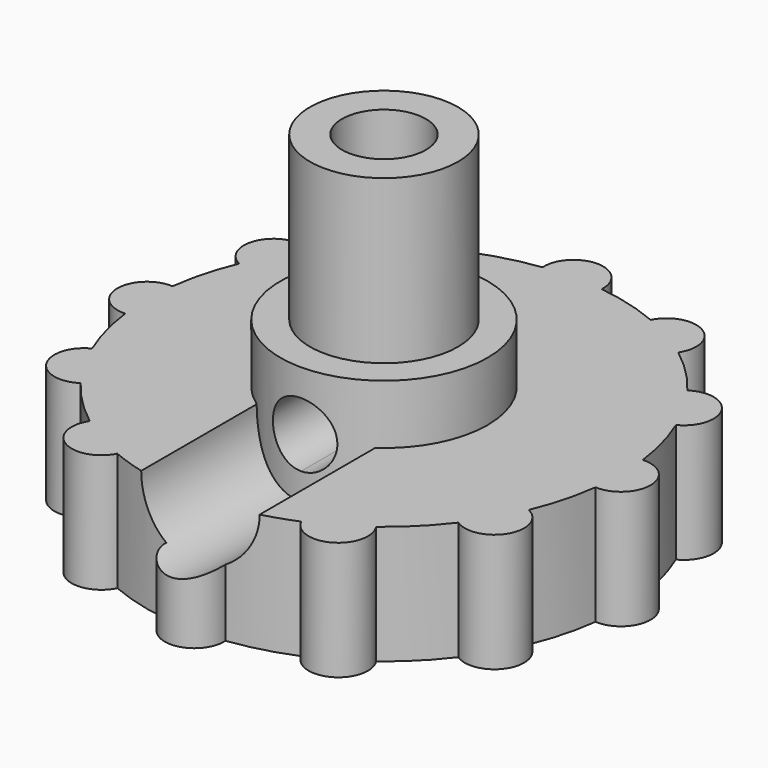
from build123d import *

# Parameters (mm, degrees)
F0_R           = 12.7
F1_DEPTH       = 6.35
F3_DEPTH       = 3.175
F4_R           = 5.55625
F5_DEPTH       = 3.175
F6_R           = 3.96875
F7_DEPTH       = 8.73125
F8_R           = 2.2479
F9_DEPTH       = 15.08125
F11_DEPTH      = 6.35
F12_COUNT      = 12
F12_ANGLE      = 330
F14_END_RADIUS = 5.55625
F14_REACH      = 18.1506366107
F17_END_RADIUS = 5.55625
F17_REACH      = 35.6755158286


with BuildPart() as f1:
    # F0 (on Top) → F1 (new body)
    with BuildSketch(Plane.XY):
        Circle(F0_R)
    extrude(amount=F1_DEPTH)

    # F2 (on face) → F3 (cut)
    with BuildSketch(Plane(origin=(0, 0, 0), x_dir=(1, 0, 0), z_dir=(0, 0, -1))):
        Polygon((2.6100007461, 4.5206539), (-2.6100007461, 4.5206539), (-5.2200014922, 0), (-2.6100007461, -4.5206539), (2.6100007461, -4.5206539), (5.2200014922, 0), align=None)
    extrude(amount=-F3_DEPTH, mode=Mode.SUBTRACT)

    # F4 (on face) → F5 (join)
    with BuildSketch(Plane.XY.offset(6.35)):
        Circle(F4_R)
    extrude(amount=F5_DEPTH)

    # F6 (on face) → F7 (join)
    with BuildSketch(Plane.XY.offset(9.525)):
        Circle(F6_R)
    extrude(amount=F7_DEPTH)

    # F8 (on face) → F9 (cut, through all)
    with BuildSketch(Plane(origin=(0, 0, 3.175), x_dir=(1, 0, 0), z_dir=(0, 0, -1))):
        Circle(F8_R)
    extrude(amount=-F9_DEPTH, mode=Mode.SUBTRACT)

    # F10 (on face) → F11 (join, through all)
    with BuildSketch(Plane(origin=(0, 0, 0), x_dir=(1, 0, 0), z_dir=(0, 0, -1))):
        with BuildLine():
            ThreePointArc((-1.5843963802, 12.60078125), (0, 12.7), (1.5843963802, 12.60078125))
            ThreePointArc((1.5843963802, 12.60078125), (0, 14.2875), (-1.5843963802, 12.60078125))
        make_face()
    f11 = extrude(amount=-F11_DEPTH)

    # F12: F11 ×12 about axis
    f12_axis = Axis((0, 0, 0), (0, 0, -1))
    for i in range(1, F12_COUNT):
        add(f11.rotate(f12_axis, i * F12_ANGLE / (F12_COUNT - 1)))

    f14_end = (Plane(origin=(0, 0, 7.9375), x_dir=(-1, 0, 0), z_dir=(0, 0, -1)) * Cylinder(F14_END_RADIUS, 124.9884067655, mode=Mode.PRIVATE)).faces().sort_by_distance((-5.55625, 0, 7.9375))[0]
    # F13 (on Front) → F14 (cut, up to the whole of a round face its end follows)
    with BuildSketch(Plane.XZ):
        with BuildLine():
            ThreePointArc((0, 8.0772), (-1.7272, 6.35), (0, 4.6228))
            Line((0, 4.6228), (0, 8.0772))
        make_face()
        with BuildLine():
            Line((0, 8.0772), (0, 4.6228))
            ThreePointArc((0, 4.6228), (1.2213148325, 5.1286851675), (1.7272, 6.35))
            ThreePointArc((1.7272, 6.35), (1.2213148325, 7.5713148325), (0, 8.0772))
        make_face()
    f14_long = extrude(amount=F14_REACH, mode=Mode.PRIVATE)
    add(split(f14_long, bisect_by=f14_end, keep=Keep.BOTTOM, mode=Mode.PRIVATE), mode=Mode.SUBTRACT)

    f17_end = (Plane(origin=(0, 0, 7.9375), x_dir=(-1, 0, 0), z_dir=(0, 0, -1)) * Cylinder(F17_END_RADIUS, 160.0381652835, mode=Mode.PRIVATE)).faces().sort_by_distance((-5.55625, 0, 7.9375))[0]
    # F16 (on offset) → F17 (cut, up to the whole of a round face its end follows)
    with BuildSketch(Plane.XZ.offset(14.2875)):
        with BuildLine():
            Line((3.175, 6.35), (-3.175, 6.35))
            ThreePointArc((-3.175, 6.35), (0, 3.175), (3.175, 6.35))
        make_face()
    f17_long = extrude(amount=-F17_REACH, mode=Mode.PRIVATE)
    add(split(f17_long, bisect_by=f17_end, keep=Keep.ALL, mode=Mode.PRIVATE).solids().sort_by_distance((0, -14.2875, 5.0024881485))[0], mode=Mode.SUBTRACT)


solid = f1.part
